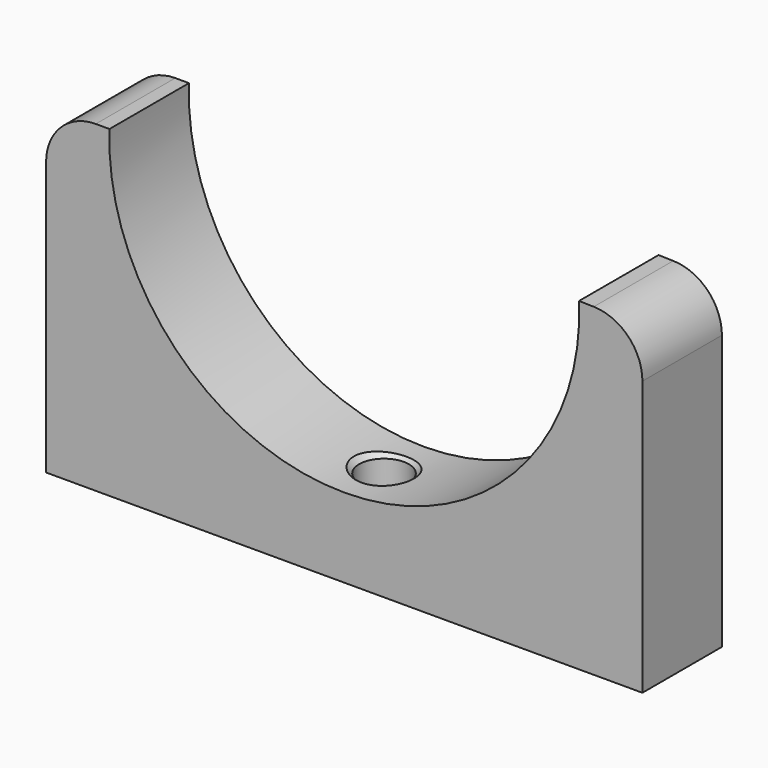
from build123d import *

# Parameters (mm, degrees)
F1_DEPTH    = 12.7
F3_R        = 4.7625
F4_DEPTH    = 6.35
F5_R        = 3.175
F6_DEPTH    = 12.7
F7_S5_R     = 30.0250138604
F7_T6_DEPTH = 8
F7_S7_R     = 3.175
F7_T8_DEPTH = 8
F8_R        = 6.35


# Not quite as in the source:
# - a fillet or chamfer that OpenCascade refuses, or shapes differently, is made with other operations: its cross-section is extruded or revolved along the edge and cut away or added


with BuildPart() as f1:
    # F0 (on Front) → F1 (new body)
    with BuildSketch(Plane.XZ):
        with BuildLine():
            Line((-38.1, 0), (-38.1, -41.275))
            Line((-38.1, -41.275), (38.1, -41.275))
            Line((38.1, -41.275), (38.1, 0))
            Line((38.1, 0), (30.0016984668, 0.169987541))
            ThreePointArc((30.0016984668, 0.169987541), (0.0893604764, -31.1423259445), (-29.9999146, 0))
            Line((-29.9999146, 0), (-38.1, 0))
        make_face()
    extrude(amount=F1_DEPTH)

    # F3 (on offset) → F4 (cut)
    with BuildSketch(Plane.XY.offset(-25.4)):
        with Locations((0, -6.35)):
            Circle(F3_R)
    extrude(amount=-F4_DEPTH, mode=Mode.SUBTRACT)

    # F5 (on face) → F6 (cut)
    with BuildSketch(Plane.XY.offset(-31.75)):
        with Locations((0, -6.35)):
            Circle(F5_R)
    extrude(amount=-F6_DEPTH, mode=Mode.SUBTRACT)

    # F7: chamfer of 1.778 on 1 edges, made by hand


with BuildPart() as f7_tool2:
    # F7_s3 → F7_t4 (revolve)
    with BuildSketch(Plane.XZ.offset(6.35)):
        Polygon((4.7625, -29.972), (2.9845, -31.75), (4.7625, -31.75), align=None)
    revolve(axis=Axis((0, -6.35, -31.75), (0, 0, 1)))

    # F7_s5 → F7_t6 (cut, symmetric)
    with BuildSketch(Plane.XZ.offset(6.3)):
        with Locations((0.0042984668, -1.1174325763)):
            Circle(F7_S5_R)
    extrude(amount=F7_T6_DEPTH, both=True, mode=Mode.SUBTRACT)

    # F7_s7 → F7_t8 (cut, symmetric)
    with BuildSketch(Plane.XY.offset(-30.9)):
        with Locations((0, -6.35)):
            Circle(F7_S7_R)
    extrude(amount=F7_T8_DEPTH, both=True, mode=Mode.SUBTRACT)


with BuildPart() as f1_1:
    add(f1.part)

    # F7_t1: union F7_tool2
    add(f7_tool2.part)

    # F8
    f8_edges = [f1_1.edges().sort_by_distance(p)[0] for p in [
        (-38.1, -6.35, 0),
        (38.1, -6.35, 0),
    ]]
    fillet(f8_edges, radius=F8_R)


solid = f1_1.part
